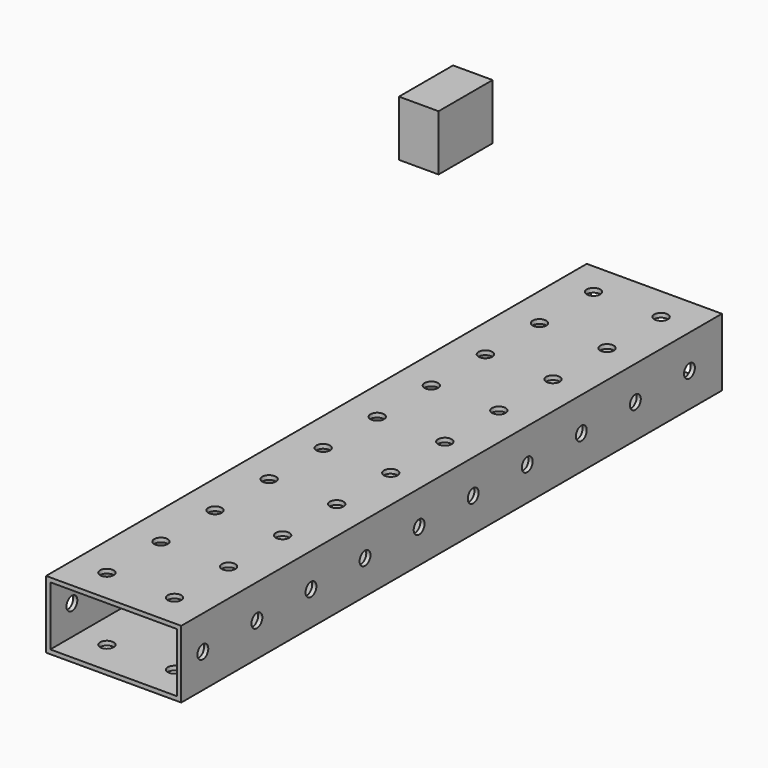
from build123d import *

# Parameters (mm, degrees)
F0_W     = 50.8
F0_H     = 25.4
F0_W_2   = 47.625
F0_H_2   = 22.225
F1_DEPTH = 254
F3_D     = 5.1054
F5_D     = 5.1054
F6_W     = 14.8742124438
F6_H     = 20.9276750684
F7_DEPTH = 25.4


# Not quite as in the source:
# - a feature names something its author has since deleted; it is built from what else it names


with BuildPart() as f1:
    # F0 (on Front) → F1 (new body)
    with BuildSketch(Plane.XZ):
        with Locations((9.4557274133, -6.3431215849)):
            Rectangle(F0_W, F0_H)
        with Locations((9.4557274133, -6.3431215849)):
            Rectangle(F0_W_2, F0_H_2, mode=Mode.SUBTRACT)
    extrude(amount=F1_DEPTH)

    # F3 (through all)
    with Locations(Plane(origin=(-15.9442725867, 0, 0), x_dir=(0, -1, 0), z_dir=(-1, 0, 0))):
        with Locations((40.6527, -6.3431215849), (66.0527, -6.3431215849), (91.4527, -6.3431215849), (116.8527, -6.3431215849), (15.2527, -6.3431215849), (142.2527, -6.3431215849), (167.6527, -6.3431215849), (193.0527, -6.3431215849), (218.4527, -6.3431215849), (243.8527, -6.3431215849)):
            Hole(F3_D / 2)

    # F5 (through all)
    with Locations(Plane(origin=(0, 0, -19.0431215849), x_dir=(1, 0, 0), z_dir=(0, 0, -1))):
        with Locations((-3.2442725867, 12.7), (22.1557274133, 12.7), (22.1557274133, 38.1), (-3.2442725867, 38.1), (22.1557274133, 63.5), (-3.2442725867, 63.5), (22.1557274133, 88.9), (-3.2442725867, 88.9), (22.1557274133, 114.3), (-3.2442725867, 114.3), (22.1557274133, 139.7), (-3.2442725867, 139.7), (22.1557274133, 165.1), (-3.2442725867, 165.1), (22.1557274133, 190.5), (-3.2442725867, 190.5), (22.1557274133, 215.9), (-3.2442725867, 215.9), (22.1557274133, 241.3), (-3.2442725867, 241.3)):
            Hole(F5_D / 2)


with BuildPart() as f7:
    # F6 (on Front) → F7 (new body)
    with BuildSketch(Plane.XZ):
        with Locations((-58.7597675622, 45.1934039593)):
            Rectangle(F6_W, F6_H)
    extrude(amount=F7_DEPTH)


solid = Compound([f1.part, f7.part])
